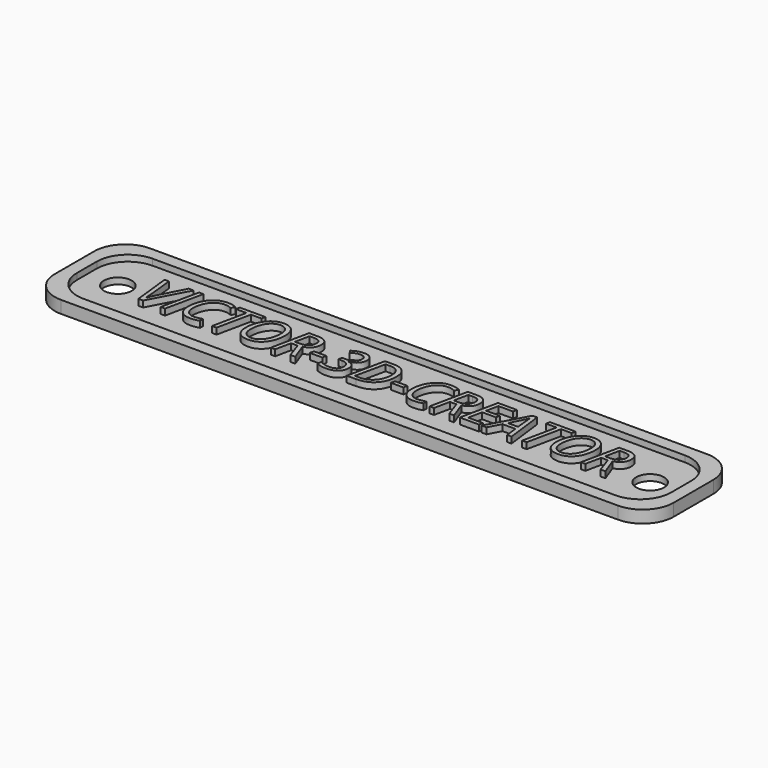
from build123d import *

# Parameters (mm, degrees)
F0_W         = 100
F0_H         = 18
F0_R         = 2.25
F1_DEPTH     = 1
F2_TEXT_SIZE = 8.5674567079
F3_DEPTH     = 1
F4_W         = 100
F4_H         = 18
F4_W_2       = 96
F4_H_2       = 14
F5_DEPTH     = 1
F6_R         = 5


# Not quite as in the source:
# - a feature names something its author has since deleted; it is built from what else it names
# - Text() gives the source's letters only with a copy of the font that has no kerning and outlines rounded to 1/6400 em; it was checked with that copy


with BuildPart() as f1:
    # F0 (on Top) → F1 (new body)
    with BuildSketch(Plane.XY):
        with Locations((50, 9)):
            Rectangle(F0_W, F0_H)
        with Locations((7, 9)):
            Circle(F0_R, mode=Mode.SUBTRACT)
        with Locations((93, 9)):
            Circle(F0_R, mode=Mode.SUBTRACT)
    extrude(amount=-F1_DEPTH)

    # F2 (on face) → F3 (join)
    with BuildSketch(Plane.XY):
        with Locations((11, 6.3314311703)):
            Text('VICTOR-3D-CREATOR', F2_TEXT_SIZE, font='Open Sans', font_style=FontStyle.ITALIC, text_align=(TextAlign.LEFT, TextAlign.BOTTOM))
    extrude(amount=F3_DEPTH)

    # F4 (on face) → F5 (join)
    with BuildSketch(Plane.XY):
        with Locations((50, 9)):
            Rectangle(F4_W, F4_H)
        with Locations((50, 9)):
            Rectangle(F4_W_2, F4_H_2, mode=Mode.SUBTRACT)
    extrude(amount=F5_DEPTH)

    # F6
    f6_edges = [f1.edges().sort_by_distance(p)[0] for p in [
        (0, 18, 0),
        (0, 0, 0),
        (100, 18, 0),
        (100, 0, 0),
        (2, 16, 0.5),
        (2, 2, 0.5),
        (98, 16, 0.5),
        (98, 2, 0.5),
    ]]
    fillet(f6_edges, radius=F6_R)


solid = f1.part
